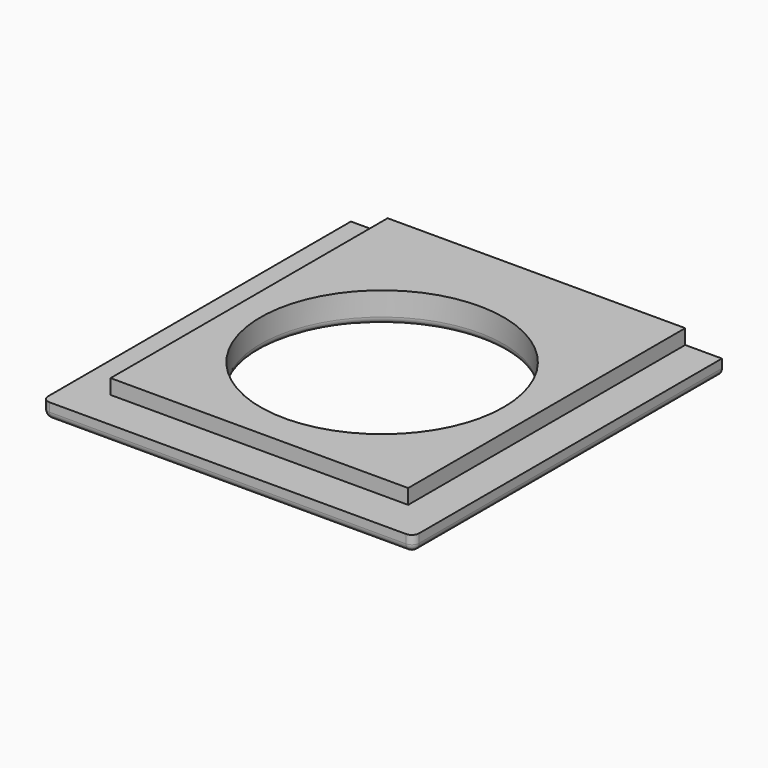
from build123d import *

# Parameters (mm, degrees)
F0_W         = 101.77
F0_H         = 105.82
F0_R         = 33.37
F1_DEPTH     = 4.38
F2_W         = 81.63
F2_H         = 94.99
F2_R         = 33.37
F3_DEPTH     = 4.07
F4_R         = 2
F5_T1_DEPTH  = 7.38
F5_S5_W      = 2
F5_S5_H      = 2
F5_T6_DEPTH  = 2
F5_S11_W     = 2
F5_S11_H     = 2
F5_T12_DEPTH = 2


# Not quite as in the source:
# - a fillet or chamfer that OpenCascade refuses, or shapes differently, is made with other operations: its cross-section is extruded or revolved along the edge and cut away or added


with BuildPart() as f1:
    # F0 (on Top) → F1 (new body)
    with BuildSketch(Plane.XY):
        Rectangle(F0_W, F0_H)
        Circle(F0_R, mode=Mode.SUBTRACT)
    extrude(amount=F1_DEPTH)

    # F2 (on face) → F3 (join)
    with BuildSketch(Plane.XY.offset(4.38)):
        with Locations((0, 5.415)):
            Rectangle(F2_W, F2_H)
        Circle(F2_R, mode=Mode.SUBTRACT)
    extrude(amount=F3_DEPTH)

    # F4
    f4_edges = [f1.edges().sort_by_distance(p)[0] for p in [
        (-33.37, 0, 0),
        (-50.885, 0, 0),
        (0, -52.91, 0),
        (50.885, 0, 0),
    ]]
    fillet(f4_edges, radius=F4_R)

    # F5: fillet of radius 2 on 2 edges, made by hand

    # F5_s2 → F5_t1 (cut)
    with BuildSketch(Plane.XY.offset(2)):
        with BuildLine():
            ThreePointArc((48.885, -52.91), (50.2992135624, -52.3242135624), (50.885, -50.91))
            Line((50.885, -50.91), (50.885, -52.91))
            Line((50.885, -52.91), (48.885, -52.91))
        make_face()
        with BuildLine():
            ThreePointArc((-48.885, -52.91), (-50.2992135624, -52.3242135624), (-50.885, -50.91))
            Line((-50.885, -50.91), (-50.885, -52.91))
            Line((-50.885, -52.91), (-48.885, -52.91))
        make_face()
    extrude(amount=F5_T1_DEPTH, mode=Mode.SUBTRACT)


with BuildPart() as f5_tool4:
    # F5_s5 → F5_t6 (new body)
    with BuildSketch(Plane.XZ.offset(50.91)):
        with Locations((-49.885, 1)):
            Rectangle(F5_S5_W, F5_S5_H)
    extrude(amount=F5_T6_DEPTH)

    # F5_s7 → F5_t8 (revolve, cut)
    with BuildSketch(Plane(origin=(-48.885, -50.91, 2), x_dir=(0.7071067812, 0, 0.7071067812), z_dir=(0.7071067812, 0, -0.7071067812))):
        with BuildLine():
            ThreePointArc((0, -2), (2, 0), (0, 2))
            Line((0, 2), (0, -2))
        make_face()
    revolve(axis=Axis((-48.885, -50.91, 2), (0, -1, 0)), mode=Mode.SUBTRACT)


with BuildPart() as f1_1:
    add(f1.part)

    # F5_t3: cut F5_tool4
    add(f5_tool4.part, mode=Mode.SUBTRACT)


with BuildPart() as f5_tool10:
    # F5_s11 → F5_t12 (new body)
    with BuildSketch(Plane.XZ.offset(50.91)):
        with Locations((49.885, 1)):
            Rectangle(F5_S11_W, F5_S11_H)
    extrude(amount=F5_T12_DEPTH)

    # F5_s13 → F5_t14 (revolve, cut)
    with BuildSketch(Plane(origin=(48.885, -50.91, 2), x_dir=(-0.7071067812, 0, 0.7071067812), z_dir=(0.7071067812, 0, 0.7071067812))):
        with BuildLine():
            ThreePointArc((0, -2), (2, 0), (0, 2))
            Line((0, 2), (0, -2))
        make_face()
    revolve(axis=Axis((48.885, -50.91, 2), (0, -1, 0)), mode=Mode.SUBTRACT)


with BuildPart() as f1_2:
    add(f1_1.part)

    # F5_t9: cut F5_tool10
    add(f5_tool10.part, mode=Mode.SUBTRACT)


solid = f1_2.part
